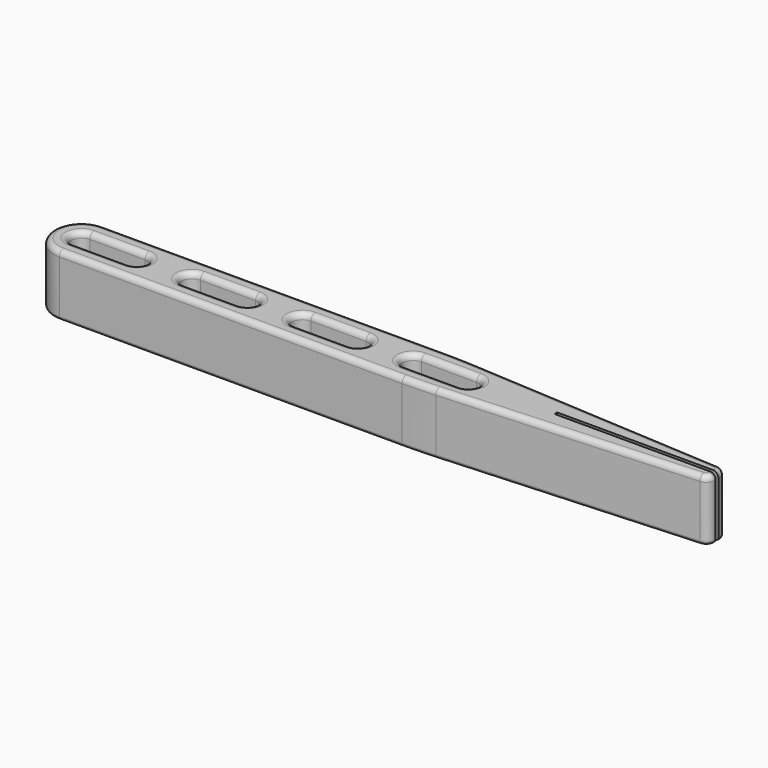
from build123d import *

# Parameters (mm, degrees)
F1_DEPTH      = 11
F2_SIZE2      = 50
F2_SIZE       = 3
F3_SIZE2      = 50
F3_SIZE       = 3
F4_R          = 1.5
F5_T1_DEPTH   = 25.9865242455
F7_DEPTH      = 25
F8_R          = 0.5
F9_R          = 1
F10_T1_DEPTH  = 11
F10_T4_ANGLE  = 90
F10_T6_ANGLE  = 90
F10_T8_ANGLE  = 90
F10_T10_ANGLE = 90


# Not quite as in the source:
# - a fillet or chamfer that OpenCascade refuses, or shapes differently, is made with other operations: its cross-section is extruded or revolved along the edge and cut away or added


with BuildPart() as f1:
    # F0 (on Top) → F1 (new body)
    with BuildSketch(Plane.XY):
        Polygon((59.5520450175, 1.9847389825), (-60.4479549825, 1.9847389825), (-60.4479549825, -8.0152610175), (59.5520450175, -8.0152610175), (59.5520450175, -3.3152610175), (30.4023410931, -3.3152610175), (30.4023410931, -2.7152610175), (59.5520450175, -2.7152610175), align=None)
    extrude(amount=F1_DEPTH)

    # F2
    f2_edges = [f1.edges().sort_by_distance(p)[0] for p in [
        (59.552045, -8.015261, 5.5),
    ]]
    f2_side = f1.faces().sort_by_distance((59.552045, -5.665261, 5.5))[0]
    chamfer(f2_edges, length=F2_SIZE, length2=F2_SIZE2, reference=f2_side)

    # F3
    f3_edges = [f1.edges().sort_by_distance(p)[0] for p in [
        (59.552045, 1.984739, 5.5),
    ]]
    f3_side = f1.faces().sort_by_distance((59.552045, -0.365261, 5.5))[0]
    chamfer(f3_edges, length=F3_SIZE, length2=F3_SIZE2, reference=f3_side)

    # F4
    f4_edges = [f1.edges().sort_by_distance(p)[0] for p in [
        (59.552045, -1.015261, 5.5),
        (59.552045, -5.015261, 5.5),
    ]]
    fillet(f4_edges, radius=F4_R)

    # F5: fillet of radius 100 on 2 edges, made by hand

    # F5_s2 → F5_t1 (cut)
    with BuildSketch(Plane.XY.offset(-7.4932621227)):
        with BuildLine():
            ThreePointArc((6.5547401684, -8.0152610175), (9.5506995592, -7.9703720791), (12.5439692412, -7.8357455641))
            Line((12.5439692412, -7.8357455641), (9.5520450175, -8.0152610175))
            Line((9.5520450175, -8.0152610175), (6.5547401684, -8.0152610175))
        make_face()
        with BuildLine():
            ThreePointArc((12.5439692412, 1.805223529), (9.5506995592, 1.939850044), (6.5547401684, 1.9847389825))
            Line((6.5547401684, 1.9847389825), (9.5520450175, 1.9847389825))
            Line((9.5520450175, 1.9847389825), (12.5439692412, 1.805223529))
        make_face()
    extrude(amount=F5_T1_DEPTH, mode=Mode.SUBTRACT)

    # F6 (on face) → F7 (cut)
    with BuildSketch(Plane.XY.offset(11)):
        with BuildLine():
            ThreePointArc((-55.4479549825, -4.9046398905), (-54.1119623692, -4.3512536308), (-53.5585761096, -3.0152610175))
            ThreePointArc((-53.5585761096, -3.0152610175), (-54.1119623692, -1.6792684042), (-55.4479549825, -1.1258821446))
            ThreePointArc((-55.4479549825, -1.1258821446), (-57.3373338555, -3.0152610175), (-55.4479549825, -4.9046398905))
        make_face()
        with BuildLine():
            ThreePointArc((-55.4479549825, -1.1258821446), (-54.1119623692, -1.6792684042), (-53.5585761096, -3.0152610175))
            ThreePointArc((-53.5585761096, -3.0152610175), (-54.1119623692, -4.3512536308), (-55.4479549825, -4.9046398905))
            Line((-55.4479549825, -4.9046398905), (-45.4479549825, -4.9046398905))
            ThreePointArc((-45.4479549825, -4.9046398905), (-47.3373338555, -3.0152610175), (-45.4479549825, -1.1258821446))
            Line((-45.4479549825, -1.1258821446), (-55.4479549825, -1.1258821446))
        make_face()
        with BuildLine():
            ThreePointArc((-43.5585761096, -3.0152610175), (-44.1119623692, -1.6792684042), (-45.4479549825, -1.1258821446))
            ThreePointArc((-45.4479549825, -1.1258821446), (-47.3373338555, -3.0152610175), (-45.4479549825, -4.9046398905))
            ThreePointArc((-45.4479549825, -4.9046398905), (-44.1119623692, -4.3512536308), (-43.5585761096, -3.0152610175))
        make_face()
        with BuildLine():
            ThreePointArc((-35.4479549825, -4.9046398905), (-34.1119623692, -4.3512536308), (-33.5585761096, -3.0152610175))
            ThreePointArc((-33.5585761096, -3.0152610175), (-34.1119623692, -1.6792684042), (-35.4479549825, -1.1258821446))
            ThreePointArc((-35.4479549825, -1.1258821446), (-37.3373338555, -3.0152610175), (-35.4479549825, -4.9046398905))
        make_face()
        with BuildLine():
            ThreePointArc((-35.4479549825, -1.1258821446), (-34.1119623692, -1.6792684042), (-33.5585761096, -3.0152610175))
            ThreePointArc((-33.5585761096, -3.0152610175), (-34.1119623692, -4.3512536308), (-35.4479549825, -4.9046398905))
            Line((-35.4479549825, -4.9046398905), (-25.4479549825, -4.9046398905))
            ThreePointArc((-25.4479549825, -4.9046398905), (-27.3373338555, -3.0152610175), (-25.4479549825, -1.1258821446))
            Line((-25.4479549825, -1.1258821446), (-35.4479549825, -1.1258821446))
        make_face()
        with BuildLine():
            ThreePointArc((-23.5585761096, -3.0152610175), (-24.1119623692, -1.6792684042), (-25.4479549825, -1.1258821446))
            ThreePointArc((-25.4479549825, -1.1258821446), (-27.3373338555, -3.0152610175), (-25.4479549825, -4.9046398905))
            ThreePointArc((-25.4479549825, -4.9046398905), (-24.1119623692, -4.3512536308), (-23.5585761096, -3.0152610175))
        make_face()
        with BuildLine():
            ThreePointArc((-15.4479549825, -4.9046398905), (-14.1119623692, -4.3512536308), (-13.5585761096, -3.0152610175))
            ThreePointArc((-13.5585761096, -3.0152610175), (-14.1119623692, -1.6792684042), (-15.4479549825, -1.1258821446))
            ThreePointArc((-15.4479549825, -1.1258821446), (-17.3373338555, -3.0152610175), (-15.4479549825, -4.9046398905))
        make_face()
        with BuildLine():
            ThreePointArc((-15.4479549825, -1.1258821446), (-14.1119623692, -1.6792684042), (-13.5585761096, -3.0152610175))
            ThreePointArc((-13.5585761096, -3.0152610175), (-14.1119623692, -4.3512536308), (-15.4479549825, -4.9046398905))
            Line((-15.4479549825, -4.9046398905), (-5.4479549825, -4.9046398905))
            ThreePointArc((-5.4479549825, -4.9046398905), (-7.3373338555, -3.0152610175), (-5.4479549825, -1.1258821446))
            Line((-5.4479549825, -1.1258821446), (-15.4479549825, -1.1258821446))
        make_face()
        with BuildLine():
            ThreePointArc((-3.5585761096, -3.0152610175), (-4.1119623692, -1.6792684042), (-5.4479549825, -1.1258821446))
            ThreePointArc((-5.4479549825, -1.1258821446), (-7.3373338555, -3.0152610175), (-5.4479549825, -4.9046398905))
            ThreePointArc((-5.4479549825, -4.9046398905), (-4.1119623692, -4.3512536308), (-3.5585761096, -3.0152610175))
        make_face()
        with BuildLine():
            ThreePointArc((4.5520450175, -4.9046398905), (5.8880376308, -4.3512536308), (6.4414238904, -3.0152610175))
            ThreePointArc((6.4414238904, -3.0152610175), (5.8880376308, -1.6792684042), (4.5520450175, -1.1258821446))
            ThreePointArc((4.5520450175, -1.1258821446), (2.6626661445, -3.0152610175), (4.5520450175, -4.9046398905))
        make_face()
        with BuildLine():
            ThreePointArc((4.5520450175, -1.1258821446), (5.8880376308, -1.6792684042), (6.4414238904, -3.0152610175))
            ThreePointArc((6.4414238904, -3.0152610175), (5.8880376308, -4.3512536308), (4.5520450175, -4.9046398905))
            Line((4.5520450175, -4.9046398905), (14.5520450175, -4.9046398905))
            ThreePointArc((14.5520450175, -4.9046398905), (12.6626661445, -3.0152610175), (14.5520450175, -1.1258821446))
            Line((14.5520450175, -1.1258821446), (4.5520450175, -1.1258821446))
        make_face()
        with BuildLine():
            ThreePointArc((16.4414238904, -3.0152610175), (15.8880376308, -1.6792684042), (14.5520450175, -1.1258821446))
            ThreePointArc((14.5520450175, -1.1258821446), (12.6626661445, -3.0152610175), (14.5520450175, -4.9046398905))
            ThreePointArc((14.5520450175, -4.9046398905), (15.8880376308, -4.3512536308), (16.4414238904, -3.0152610175))
        make_face()
    extrude(amount=-F7_DEPTH, mode=Mode.SUBTRACT)

    # F8
    f8_edges = [f1.edges().sort_by_distance(p)[0] for p in [
        (35.342926, -6.467808, 0),
        (9.5507, 1.93985, 0),
        (-60.447955, -3.015261, 0),
        (-43.558576, -3.015261, 0),
        (-23.558576, -3.015261, 0),
        (-3.558576, -3.015261, 0),
        (16.441424, -3.015261, 0),
    ]]
    fillet(f8_edges, radius=F8_R)

    # F9
    f9_edges = [f1.edges().sort_by_distance(p)[0] for p in [
        (-26.946607, 1.984739, 11),
        (-26.946607, -8.015261, 11),
        (-60.447955, -3.015261, 11),
        (-43.558576, -3.015261, 11),
        (-23.558576, -3.015261, 11),
        (-3.558576, -3.015261, 11),
        (16.441424, -3.015261, 11),
    ]]
    fillet(f9_edges, radius=F9_R)

    # F10: fillet of radius 5 on 2 edges, made by hand

    # F10_s2 → F10_t1 (cut)
    with BuildSketch(Plane.XY):
        with BuildLine():
            ThreePointArc((-55.4479549825, 1.9847389825), (-58.9834888885, 0.5202728884), (-60.4479549825, -3.0152610175))
            Line((-60.4479549825, -3.0152610175), (-60.4479549825, 1.9847389825))
            Line((-60.4479549825, 1.9847389825), (-55.4479549825, 1.9847389825))
        make_face()
        with BuildLine():
            ThreePointArc((-60.4479549825, -3.0152610175), (-58.9834888885, -6.5507949235), (-55.4479549825, -8.0152610175))
            Line((-55.4479549825, -8.0152610175), (-60.4479549825, -8.0152610175))
            Line((-60.4479549825, -8.0152610175), (-60.4479549825, -3.0152610175))
        make_face()
    extrude(amount=F10_T1_DEPTH, mode=Mode.SUBTRACT)

    # F10_s3 → F10_t4 (revolve, cut)
    with BuildSketch(Plane.YZ.offset(-55.4479549825)):
        with BuildLine():
            ThreePointArc((-7.5152610175, 0), (-7.8688144081, 0.1464466094), (-8.0152610175, 0.5))
            Line((-8.0152610175, 0.5), (-8.0152610175, 0))
            Line((-8.0152610175, 0), (-7.5152610175, 0))
        make_face()
    revolve(axis=Axis((-55.4479549825, -3.0152610175, 0), (0, 0, -1)), revolution_arc=F10_T4_ANGLE, mode=Mode.SUBTRACT)

    # F10_s5 → F10_t6 (revolve, cut)
    with BuildSketch(Plane.XZ.offset(3.0152610175)):
        with BuildLine():
            ThreePointArc((-59.4479549825, 11), (-60.1550617637, 10.7071067812), (-60.4479549825, 10))
            Line((-60.4479549825, 10), (-60.4479549825, 11))
            Line((-60.4479549825, 11), (-59.4479549825, 11))
        make_face()
    revolve(axis=Axis((-55.4479549825, -3.0152610175, 11), (0, 0, 1)), revolution_arc=F10_T6_ANGLE, mode=Mode.SUBTRACT)

    # F10_s7 → F10_t8 (revolve, cut)
    with BuildSketch(Plane.XZ.offset(3.0152610175)):
        with BuildLine():
            ThreePointArc((-59.9479549825, 0), (-60.3015083731, 0.1464466094), (-60.4479549825, 0.5))
            Line((-60.4479549825, 0.5), (-60.4479549825, 0))
            Line((-60.4479549825, 0), (-59.9479549825, 0))
        make_face()
    revolve(axis=Axis((-55.4479549825, -3.0152610175, 0), (0, 0, -1)), revolution_arc=F10_T8_ANGLE, mode=Mode.SUBTRACT)

    # F10_s9 → F10_t10 (revolve, cut)
    with BuildSketch(Plane.YZ.offset(-55.4479549825)):
        with BuildLine():
            ThreePointArc((0.9847389825, 11), (1.6918457637, 10.7071067812), (1.9847389825, 10))
            Line((1.9847389825, 10), (1.9847389825, 11))
            Line((1.9847389825, 11), (0.9847389825, 11))
        make_face()
    revolve(axis=Axis((-55.4479549825, -3.0152610175, 11), (0, 0, 1)), revolution_arc=F10_T10_ANGLE, mode=Mode.SUBTRACT)


solid = f1.part
